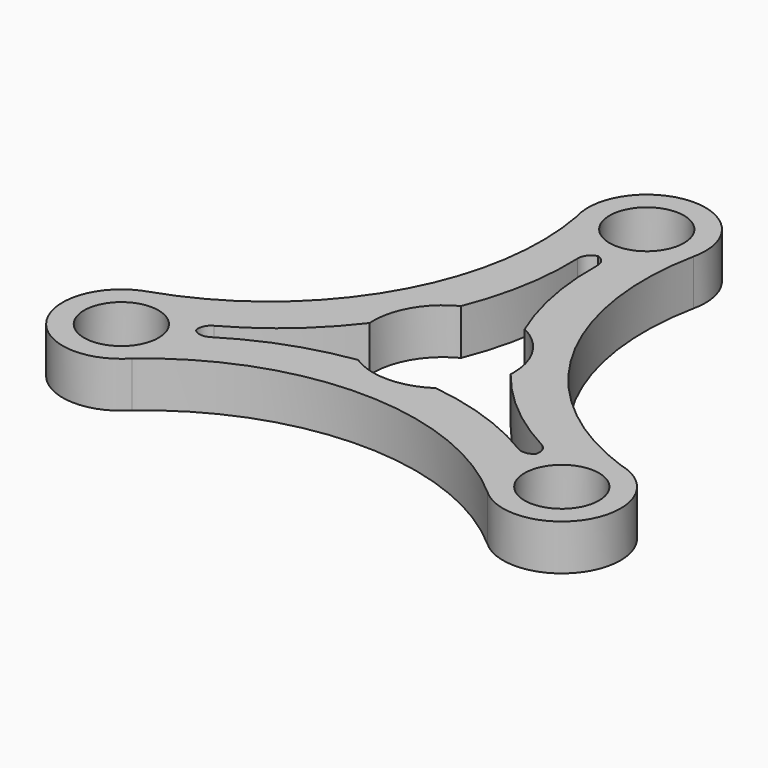
from build123d import *

# Parameters (mm, degrees)
F0_R        = 5.7
F1_DEPTH    = 7
F2_T1_DEPTH = 7


# Not quite as in the source:
# - a fillet or chamfer that OpenCascade refuses, or shapes differently, is made with other operations: its cross-section is extruded or revolved along the edge and cut away or added


with BuildPart() as f1:
    # F0 (on Top) → F1 (new body)
    with BuildSketch(Plane.XY):
        with BuildLine():
            ThreePointArc((35.7857254885, -10.7114257283), (13.3672908486, 8.0601420356), (8.7727432709, 36.9365701488))
            ThreePointArc((8.7727432709, 36.9365701488), (-0.3049324387, 47.9411231542), (-8.6164959528, 36.3470602301))
            ThreePointArc((-8.6164959528, 36.3470602301), (-13.6639331853, 7.5463424369), (-36.374379713, -10.8708665409))
            ThreePointArc((-36.374379713, -10.8708665409), (-41.3657643181, -24.2346408155), (-27.1692295357, -25.6356345017))
            ThreePointArc((-27.1692295357, -25.6356345017), (0.2966423367, -15.6064844725), (27.6016364421, -26.0657036079))
            ThreePointArc((27.6016364421, -26.0657036079), (41.6706967568, -23.7064823387), (35.7857254885, -10.7114257283))
        make_face()
        with Locations((-33.7284768728, -19.4731452019)):
            Circle(F0_R, mode=Mode.SUBTRACT)
        with Locations((33.7284768728, -19.4731452019)):
            Circle(F0_R, mode=Mode.SUBTRACT)
        with BuildLine():
            ThreePointArc((4.7464996897, 9.6453740568), (9.1265374503, 5.6805645994), (10.75, 0))
            ThreePointArc((10.75, 0), (10.7467864276, -0.2628335582), (10.7371476318, -0.5255099751))
            ThreePointArc((10.7371476318, -0.5255099751), (18.1244877352, -7.9521533479), (27.0404212358, -13.4506945549))
            ThreePointArc((27.0404212358, -13.4506945549), (26.0732155549, -14.7406010495), (25.3516724639, -16.1823781342))
            ThreePointArc((25.3516724639, -16.1823781342), (16.0918632419, -11.4192065952), (5.9798891173, -8.9332763388))
            ThreePointArc((5.9798891173, -8.9332763388), (0.0934488338, -10.749593821), (-5.8236788043, -9.0358876257))
            ThreePointArc((-5.8236788043, -9.0358876257), (-15.9490106817, -11.7201901353), (-25.168853801, -16.6923444418))
            ThreePointArc((-25.168853801, -16.6923444418), (-25.8023427534, -15.2097665041), (-26.6901867898, -13.864003315))
            ThreePointArc((-26.6901867898, -13.864003315), (-17.9352546235, -8.2263590641), (-10.726388807, -0.712097718))
            ThreePointArc((-10.726388807, -0.712097718), (-9.3561457462, 5.2938678465), (-4.9134688275, 9.5613976008))
            ThreePointArc((-4.9134688275, 9.5613976008), (-2.1754770535, 19.6723434832), (-1.8715674348, 30.1430389967))
            ThreePointArc((-1.8715674348, 30.1430389967), (-0.2708728015, 29.9503675537), (1.3385143259, 30.0463814492))
            ThreePointArc((1.3385143259, 30.0463814492), (1.8433913815, 19.6455656593), (4.7464996897, 9.6453740568))
        make_face(mode=Mode.SUBTRACT)
        with Locations((0, 38.9462904038)):
            Circle(F0_R, mode=Mode.SUBTRACT)
    extrude(amount=F1_DEPTH)

    # F2: fillet of radius 2 on 6 edges, made by hand

    # F2_s2 → F2_t1 (join)
    with BuildSketch(Plane.XY):
        with BuildLine():
            ThreePointArc((1.2437301381, 27.9302712072), (0.7204204263, 29.321617428), (-0.6184050998, 29.9675613661))
            ThreePointArc((-0.6184050998, 29.9675613661), (0.362205019, 29.9535818283), (1.3385143259, 30.0463814492))
            ThreePointArc((1.3385143259, 30.0463814492), (1.278556326, 28.9888891766), (1.2437301381, 27.9302712072))
        make_face()
        with BuildLine():
            ThreePointArc((0.2214111543, 29.9490143104), (-1.1869742591, 29.3190857733), (-1.7279638998, 27.8742018185))
            ThreePointArc((-1.7279638998, 27.8742018185), (-1.7853057388, 29.0095356327), (-1.8715674348, 30.1430389967))
            ThreePointArc((-1.8715674348, 30.1430389967), (-0.8307618987, 29.984714947), (0.2214111543, 29.9490143104))
        make_face()
        with BuildLine():
            ThreePointArc((23.566459331, -15.0422374987), (25.0330553595, -15.2847111045), (26.2618719824, -14.4482261568))
            ThreePointArc((26.2618719824, -14.4482261568), (25.7594602881, -15.290469662), (25.3516724639, -16.1823781342))
            ThreePointArc((25.3516724639, -16.1823781342), (24.4658362914, -15.6017068468), (23.566459331, -15.0422374987))
        make_face()
        with BuildLine():
            ThreePointArc((25.825901634, -15.1662548395), (25.9845602249, -13.6315930247), (25.0037488349, -12.4406402752))
            ThreePointArc((25.0037488349, -12.4406402752), (26.0156476793, -12.958647693), (27.0404212358, -13.4506945549))
            ThreePointArc((27.0404212358, -13.4506945549), (26.3829058187, -14.2728965647), (25.825901634, -15.1662548395))
        make_face()
        with BuildLine():
            ThreePointArc((-25.6434668826, -15.5193352093), (-25.7534757858, -14.0369063234), (-24.8101894691, -12.8880337086))
            ThreePointArc((-24.8101894691, -12.8880337086), (-25.7443926174, -13.3871823298), (-26.6901867898, -13.864003315))
            ThreePointArc((-26.6901867898, -13.864003315), (-26.1216653071, -14.6631121663), (-25.6434668826, -15.5193352093))
        make_face()
        with BuildLine():
            ThreePointArc((-26.0473127882, -14.7827594709), (-24.7975859659, -15.6874927486), (-23.2757849351, -15.4335615433))
            ThreePointArc((-23.2757849351, -15.4335615433), (-24.2303419405, -16.0508879397), (-25.168853801, -16.6923444418))
            ThreePointArc((-25.168853801, -16.6923444418), (-25.55214392, -15.7118183822), (-26.0473127882, -14.7827594709))
        make_face()
    extrude(amount=F2_T1_DEPTH)


solid = f1.part
